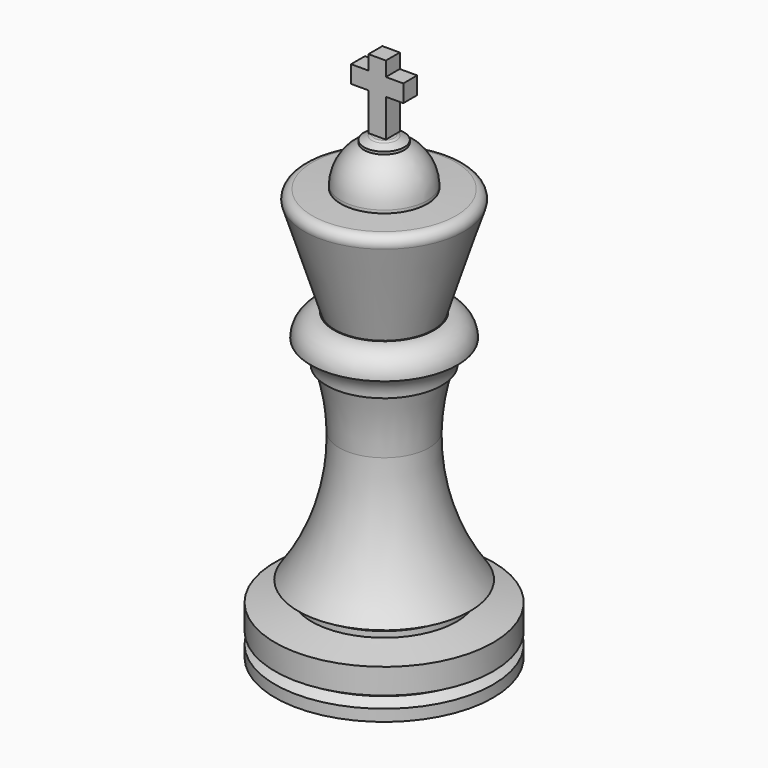
from build123d import *

# Parameters (mm, degrees)
F0_W     = 12.5
F0_H     = 1
F3_DEPTH = 1.5


# Not quite as in the source:
# - a feature names something its author has since deleted; it is built from what else it names


with BuildPart() as f1:
    # F0 (on Front) → F1 (revolve)
    with BuildSketch(Plane.XZ):
        Polygon((18.8, 0), (18.8, 2.0002274268), (17.0679491924, 3.0002274268), (18.8, 4.0002274268), (18.8, 8.3626933041), (12.5, 9.5), (0, 9.5), (0, 1.2), (16.35, 1.2), (16.35, 0), align=None)
        with Locations((6.25, 10)):
            Rectangle(F0_W, F0_H)
        with BuildLine():
            Line((0, 34.3426428735), (7.75, 34.3426428735))
            ThreePointArc((7.75, 34.3426428735), (8.2028205644, 39.4771439193), (9.36, 44.5))
            Line((9.36, 44.5), (0, 44.5))
            Line((0, 44.5), (0, 34.3426428735))
        make_face()
        with BuildLine():
            Line((0, 44.5), (9.36, 44.5))
            Line((9.36, 44.5), (9.9101864842, 44.5))
            ThreePointArc((9.9101864842, 44.5), (10.6608114666, 46.9241791446), (12.65, 48.5))
            Line((12.65, 48.5), (8.65, 48.5))
            Line((8.65, 48.5), (0, 48.5))
            Line((0, 48.5), (0, 44.5))
        make_face()
        with BuildLine():
            Line((8.65, 48.5), (12.65, 48.5))
            ThreePointArc((12.65, 48.5), (11.4784271247, 51.3284271247), (8.65, 52.5))
            Line((8.65, 52.5), (8.65, 48.5))
        make_face()
        with BuildLine():
            Line((0, 10.5), (12.5, 10.5))
            Line((12.5, 10.5), (14.8, 11.8279056191))
            ThreePointArc((14.8, 11.8279056191), (9.4456568695, 22.5124552556), (7.75, 34.3426428735))
            Line((7.75, 34.3426428735), (0, 34.3426428735))
            Line((0, 34.3426428735), (0, 10.5))
        make_face()
    revolve(axis=Axis((0, 0, 39.4972705525), (0, 0, -1)))


with BuildPart() as f1b:
    # F0 (on Front) → F1, piece 2 (revolve)
    with BuildSketch(Plane.XZ):
        with BuildLine():
            Line((0, 64.2382279038), (0, 52.5))
            Line((0, 52.5), (8.5, 52.5))
            Line((8.5, 52.5), (13.7947297094, 69.1527789248))
            ThreePointArc((13.7947297094, 69.1527789248), (13.5912487708, 70.4715238313), (12.417594041, 71.1063680609))
            Line((12.417594041, 71.1063680609), (7.45, 71.2798402673))
            Line((7.45, 71.2798402673), (7.45, 64.2382279038))
            Line((7.45, 64.2382279038), (0, 64.2382279038))
        make_face()
        with BuildLine():
            Line((0, 78.1429223141), (0, 64.2382279038))
            Line((0, 64.2382279038), (7.45, 64.2382279038))
            Line((7.45, 64.2382279038), (7.45, 71.2798402673))
            Line((7.45, 71.2798402673), (7.45, 71.8001597327))
            ThreePointArc((7.45, 71.8001597327), (6.3098878192, 75.5093196892), (3.46, 78.1429223141))
            Line((3.46, 78.1429223141), (2.15, 78.1429223141))
            Line((2.15, 78.1429223141), (0, 78.1429223141))
        make_face()
        Polygon((0, 78.994541105), (0, 78.1429223141), (2.15, 78.1429223141), (2.15, 79.1970730977), (1.73, 79.3929223141), (0, 79.3929223141), align=None)
        Polygon((2.15, 79.1970730977), (2.15, 78.1429223141), (3.46, 78.1429223141), (3.46, 78.5862100655), align=None)
    revolve(axis=Axis((0, 0, 39.4972705525), (0, 0, -1)))


with BuildPart() as f3:
    # F2 (on Front) → F3 (new body, symmetric)
    with BuildSketch(Plane.XZ):
        Polygon((1.5, 91.7148197889), (0, 91.7148197889), (-1.5, 91.7148197889), (-1.5, 89.2148197889), (-4.5, 89.2148197889), (-4.5, 86.2148197889), (-1.5, 86.2148197889), (-1.5, 79.7148197889), (0, 79.7148197889), (1.5, 79.7148197889), (1.5, 86.2148197889), (4.5, 86.2148197889), (4.5, 89.2148197889), (1.5, 89.2148197889), align=None)
    extrude(amount=F3_DEPTH, both=True)


solid = Compound([f1.part, f1b.part, f3.part])
